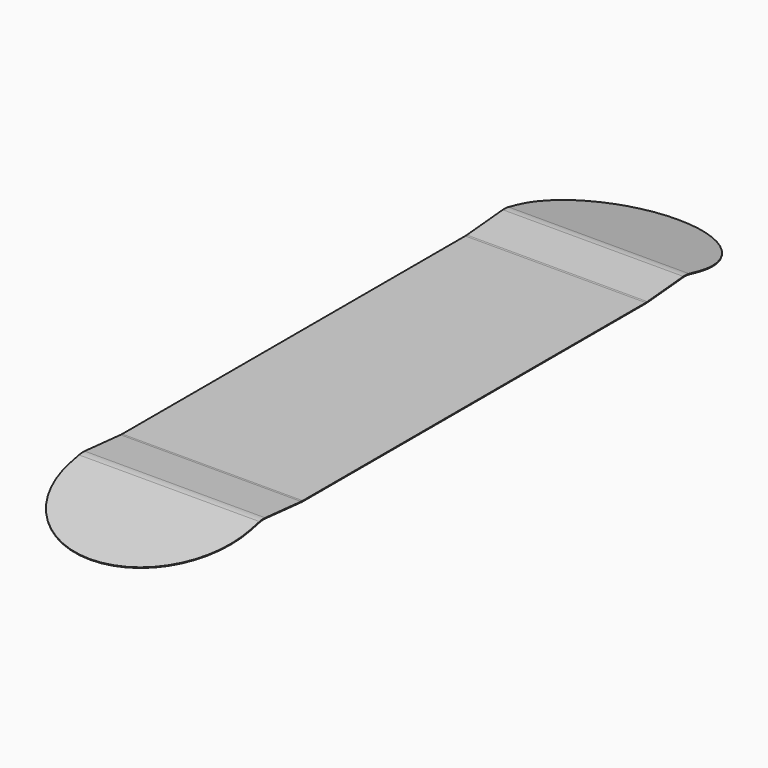
from build123d import *

# Parameters (mm, degrees)
F0_W     = 203.2
F0_H     = 482.6
F1_DEPTH = 0.79375
F3_DEPTH = 203.2
F4_R     = 101.59999


# Not quite as in the source:
# - a fillet or chamfer is up to 0.001 mm smaller than in the source, because OpenCascade refuses the exact size


with BuildPart() as f1:
    # F0 (on Top) → F1 (new body)
    with BuildSketch(Plane.XY):
        Rectangle(F0_W, F0_H)
    extrude(amount=F1_DEPTH)

    # F2 (on face) → F3 (join, through all)
    with BuildSketch(Plane.YZ.offset(101.6)):
        with BuildLine():
            ThreePointArc((243.5137558658, 0.8904046685), (242.4079324391, 0.8179251718), (241.3, 0.79375))
            Line((241.3, 0.79375), (241.3, 0))
            ThreePointArc((241.3, 0), (242.4425553278, 0.0249306459), (243.5829357366, 0.0996751269))
            Line((243.5829357366, 0.0996751269), (294.1896263997, 4.5271868584))
            ThreePointArc((294.1896263997, 4.5271868584), (298.0689507117, 4.5691740706), (301.9094190229, 4.0198807111))
            Line((301.9094190229, 4.0198807111), (413.4915953519, -20.7572846976))
            Line((413.4915953519, -20.7572846976), (413.6636590006, -19.9824084731))
            Line((413.6636590006, -19.9824084731), (302.0814826716, 4.7947569356))
            ThreePointArc((302.0814826716, 4.7947569356), (298.1209997257, 5.3612157126), (294.1204465289, 5.3179164001))
            Line((294.1204465289, 5.3179164001), (243.5137558658, 0.8904046685))
        make_face()
        with BuildLine():
            Line((-241.3, 0), (-241.3, 0.79375))
            ThreePointArc((-241.3, 0.79375), (-242.4079324391, 0.8179251718), (-243.5137558658, 0.8904046685))
            Line((-243.5137558658, 0.8904046685), (-294.1204465289, 5.3179164001))
            ThreePointArc((-294.1204465289, 5.3179164001), (-298.1209997257, 5.3612157126), (-302.0814826716, 4.7947569356))
            Line((-302.0814826716, 4.7947569356), (-413.6636590006, -19.9824084731))
            Line((-413.6636590006, -19.9824084731), (-413.4915953519, -20.7572846976))
            Line((-413.4915953519, -20.7572846976), (-301.9094190229, 4.0198807111))
            ThreePointArc((-301.9094190229, 4.0198807111), (-298.0689507117, 4.5691740706), (-294.1896263997, 4.5271868584))
            Line((-294.1896263997, 4.5271868584), (-243.5829357366, 0.0996751269))
            ThreePointArc((-243.5829357366, 0.0996751269), (-242.4425553278, 0.0249306459), (-241.3, 0))
        make_face()
    extrude(amount=-F3_DEPTH)

    # F4 (radius 101.6 in the source; OpenCascade refuses exactly that, so slightly less here)
    f4_edges = [f1.edges().sort_by_distance(p)[0] for p in [
        (101.6, 413.577627, -20.369847),
        (-101.6, 413.577627, -20.369847),
        (101.6, -413.577627, -20.369847),
        (-101.6, -413.577627, -20.369847),
    ]]
    fillet(f4_edges, radius=F4_R)


solid = f1.part
